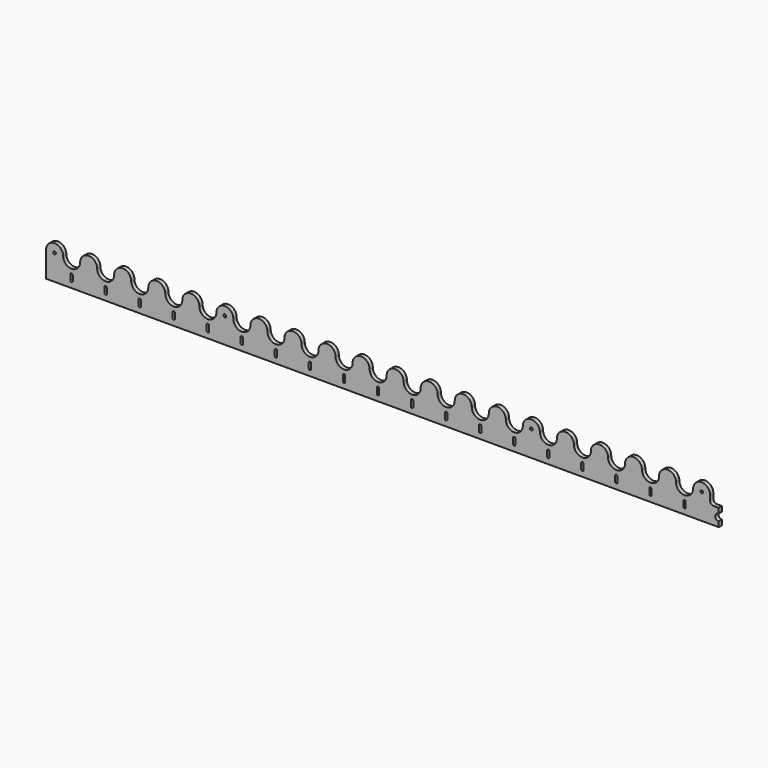
from build123d import *

# Parameters (mm, degrees)
F0_R     = 4
F1_DEPTH = 12


# Not quite as in the source:
# - ends of sketch curves that miss each other by under 0.0002 mm in the source are joined


with BuildPart() as f1:
    # F0 (on Front) → F1 (new body)
    with BuildSketch(Plane.XZ):
        with BuildLine():
            ThreePointArc((91.0431935055, 71.2102863897), (66.0431935055, 96.2102863897), (41.0431935055, 71.2102863897))
            ThreePointArc((41.0431935055, 71.2102863897), (16.0431935055, 46.2102863897), (-8.9568064945, 71.2102863897))
            ThreePointArc((-8.9568064945, 71.2102863897), (-33.9568064945, 96.2102863897), (-58.9568064945, 71.2102863897))
            Line((-58.9568064945, 71.2102863897), (-58.9568064945, -3.7897136103))
            Line((-58.9568064945, -3.7897136103), (1891.0431935055, -3.7897136103))
            Line((1891.0431935055, -3.7897136103), (1916.0431861877, -3.7897136103))
            Line((1916.0431861877, -3.7897136103), (1916.0431861877, 11.2232529739))
            ThreePointArc((1916.0431861877, 11.2232529739), (1906.0431861877, 21.2232529739), (1916.0431861877, 31.2232529739))
            Line((1916.0431861877, 31.2232529739), (1916.0431861877, 46.2362195582))
            Line((1916.0431861877, 46.2362195582), (1901.0431884565, 46.2362195582))
            ThreePointArc((1901.0431884565, 46.2362195582), (1893.9756743288, 49.1615998472), (1891.0431935055, 56.2261707472))
            Line((1891.0431935055, 56.2261707472), (1891.0431935055, 56.4615577459))
            Line((1891.0431935055, 56.4615577459), (1891.0431935055, 71.2102863897))
            ThreePointArc((1891.0431935055, 71.2102863897), (1866.0431935055, 96.2102863897), (1841.0431935055, 71.2102863897))
            ThreePointArc((1841.0431935055, 71.2102863897), (1816.0431935055, 46.2102863897), (1791.0431935055, 71.2102863897))
            ThreePointArc((1791.0431935055, 71.2102863897), (1766.0431935055, 96.2102863897), (1741.0431935055, 71.2102863897))
            ThreePointArc((1741.0431935055, 71.2102863897), (1716.0431935055, 46.2102863897), (1691.0431935055, 71.2102863897))
            ThreePointArc((1691.0431935055, 71.2102863897), (1666.0431935055, 96.2102863897), (1641.0431935055, 71.2102863897))
            ThreePointArc((1641.0431935055, 71.2102863897), (1616.0431935055, 46.2102863897), (1591.0431935055, 71.2102863897))
            ThreePointArc((1591.0431935055, 71.2102863897), (1566.0431935055, 96.2102863897), (1541.0431935055, 71.2102863897))
            ThreePointArc((1541.0431935055, 71.2102863897), (1516.0431935055, 46.2102863897), (1491.0431935055, 71.2102863897))
            ThreePointArc((1491.0431935055, 71.2102863897), (1466.0431935055, 96.2102863897), (1441.0431935055, 71.2102863897))
            ThreePointArc((1441.0431935055, 71.2102863897), (1416.0431935055, 46.2102863897), (1391.0431935055, 71.2102863897))
            ThreePointArc((1391.0431935055, 71.2102863897), (1366.0431935055, 96.2102863897), (1341.0431935055, 71.2102863897))
            ThreePointArc((1341.0431935055, 71.2102863897), (1316.0431935055, 46.2102863897), (1291.0431935055, 71.2102863897))
            ThreePointArc((1291.0431935055, 71.2102863897), (1266.0431935055, 96.2102863897), (1241.0431935055, 71.2102863897))
            ThreePointArc((1241.0431935055, 71.2102863897), (1216.0431935055, 46.2102863897), (1191.0431935055, 71.2102863897))
            ThreePointArc((1191.0431935055, 71.2102863897), (1166.0431935055, 96.2102863897), (1141.0431935055, 71.2102863897))
            ThreePointArc((1141.0431935055, 71.2102863897), (1116.0431935055, 46.2102863897), (1091.0431935055, 71.2102863897))
            ThreePointArc((1091.0431935055, 71.2102863897), (1066.0431935055, 96.2102863897), (1041.0431935055, 71.2102863897))
            ThreePointArc((1041.0431935055, 71.2102863897), (1016.0431935055, 46.2102863897), (991.0431935055, 71.2102863897))
            ThreePointArc((991.0431935055, 71.2102863897), (966.0431935055, 96.2102863897), (941.0431935055, 71.2102863897))
            ThreePointArc((941.0431935055, 71.2102863897), (916.0431935055, 46.2102863897), (891.0431935055, 71.2102863897))
            ThreePointArc((891.0431935055, 71.2102863897), (866.0431935055, 96.2102863897), (841.0431935055, 71.2102863897))
            ThreePointArc((841.0431935055, 71.2102863897), (816.0431935055, 46.2102863897), (791.0431935055, 71.2102863897))
            ThreePointArc((791.0431935055, 71.2102863897), (766.0431935055, 96.2102863897), (741.0431935055, 71.2102863897))
            ThreePointArc((741.0431935055, 71.2102863897), (716.0431935055, 46.2102863897), (691.0431935055, 71.2102863897))
            ThreePointArc((691.0431935055, 71.2102863897), (666.0431935055, 96.2102863897), (641.0431935055, 71.2102863897))
            ThreePointArc((641.0431935055, 71.2102863897), (616.0431935055, 46.2102863897), (591.0431935055, 71.2102863897))
            ThreePointArc((591.0431935055, 71.2102863897), (566.0431935055, 96.2102863897), (541.0431935055, 71.2102863897))
            ThreePointArc((541.0431935055, 71.2102863897), (516.0431935055, 46.2102863897), (491.0431935055, 71.2102863897))
            ThreePointArc((491.0431935055, 71.2102863897), (466.0431935055, 96.2102863897), (441.0431935055, 71.2102863897))
            ThreePointArc((441.0431935055, 71.2102863897), (416.0431935055, 46.2102863897), (391.0431935055, 71.2102863897))
            ThreePointArc((391.0431935055, 71.2102863897), (366.0431935055, 96.2102863897), (341.0431935055, 71.2102863897))
            ThreePointArc((341.0431935055, 71.2102863897), (316.0431935055, 46.2102863897), (291.0431935055, 71.2102863897))
            ThreePointArc((291.0431935055, 71.2102863897), (266.0431935055, 96.2102863897), (241.0431935055, 71.2102863897))
            ThreePointArc((241.0431935055, 71.2102863897), (216.0431935055, 46.2102863897), (191.0431935055, 71.2102863897))
            ThreePointArc((191.0431935055, 71.2102863897), (166.0431935055, 96.2102863897), (141.0431935055, 71.2102863897))
            ThreePointArc((141.0431935055, 71.2102863897), (116.0431935055, 46.2102863897), (91.0431935055, 71.2102863897))
        make_face()
        with BuildLine():
            ThreePointArc((12.3674108083, 31.0259666217), (15.8490323457, 34.5622976712), (19.3672217487, 31.0623449364))
            Line((19.3672217487, 31.0623449364), (19.3672217487, 14.9847705892))
            ThreePointArc((19.3672217487, 14.9847705892), (15.8854111516, 11.4848178545), (12.3674108083, 14.9483922746))
            Line((12.3674108083, 14.9483922746), (12.3674108083, 31.0259666217))
        make_face(mode=Mode.SUBTRACT)
        with BuildLine():
            Line((112.3674108083, 14.9483922746), (112.3674108083, 31.0259666217))
            ThreePointArc((112.3674108083, 31.0259666217), (115.8490323457, 34.5622976712), (119.3672217487, 31.0623449364))
            Line((119.3672217487, 31.0623449364), (119.3672217487, 14.9847705892))
            ThreePointArc((119.3672217487, 14.9847705892), (115.8854111516, 11.4848178545), (112.3674108083, 14.9483922746))
        make_face(mode=Mode.SUBTRACT)
        with BuildLine():
            Line((212.3674108083, 14.9483922746), (212.3674108083, 31.0259666217))
            ThreePointArc((212.3674108083, 31.0259666217), (215.8490323457, 34.5622976712), (219.3672217487, 31.0623449364))
            Line((219.3672217487, 31.0623449364), (219.3672217487, 14.9847705892))
            ThreePointArc((219.3672217487, 14.9847705892), (215.8854111516, 11.4848178545), (212.3674108083, 14.9483922746))
        make_face(mode=Mode.SUBTRACT)
        with BuildLine():
            Line((312.3674108083, 14.9483922746), (312.3674108083, 31.0259666217))
            ThreePointArc((312.3674108083, 31.0259666217), (315.8490323457, 34.5622976712), (319.3672217487, 31.0623449364))
            Line((319.3672217487, 31.0623449364), (319.3672217487, 14.9847705892))
            ThreePointArc((319.3672217487, 14.9847705892), (315.8854111516, 11.4848178545), (312.3674108083, 14.9483922746))
        make_face(mode=Mode.SUBTRACT)
        with BuildLine():
            Line((412.3674108083, 14.9483922746), (412.3674108083, 31.0259666217))
            ThreePointArc((412.3674108083, 31.0259666217), (415.8490323457, 34.5622976712), (419.3672217487, 31.0623449364))
            Line((419.3672217487, 31.0623449364), (419.3672217487, 14.9847705892))
            ThreePointArc((419.3672217487, 14.9847705892), (415.8854111516, 11.4848178545), (412.3674108083, 14.9483922746))
        make_face(mode=Mode.SUBTRACT)
        with BuildLine():
            Line((512.3674108083, 14.9483922746), (512.3674108083, 31.0259666217))
            ThreePointArc((512.3674108083, 31.0259666217), (515.8490323457, 34.5622976712), (519.3672217487, 31.0623449364))
            Line((519.3672217487, 31.0623449364), (519.3672217487, 14.9847705892))
            ThreePointArc((519.3672217487, 14.9847705892), (515.8854111516, 11.4848178545), (512.3674108083, 14.9483922746))
        make_face(mode=Mode.SUBTRACT)
        with BuildLine():
            Line((612.3674108083, 14.9483922746), (612.3674108083, 31.0259666217))
            ThreePointArc((612.3674108083, 31.0259666217), (615.8490323457, 34.5622976712), (619.3672217487, 31.0623449364))
            Line((619.3672217487, 31.0623449364), (619.3672217487, 14.9847705892))
            ThreePointArc((619.3672217487, 14.9847705892), (615.8854111516, 11.4848178545), (612.3674108083, 14.9483922746))
        make_face(mode=Mode.SUBTRACT)
        with BuildLine():
            Line((712.3674108083, 14.9483922746), (712.3674108083, 31.0259666217))
            ThreePointArc((712.3674108083, 31.0259666217), (715.8490323457, 34.5622976712), (719.3672217487, 31.0623449364))
            Line((719.3672217487, 31.0623449364), (719.3672217487, 14.9847705892))
            ThreePointArc((719.3672217487, 14.9847705892), (715.8854111516, 11.4848178545), (712.3674108083, 14.9483922746))
        make_face(mode=Mode.SUBTRACT)
        with BuildLine():
            Line((812.3674108083, 14.9483922746), (812.3674108083, 31.0259666217))
            ThreePointArc((812.3674108083, 31.0259666217), (815.8490323457, 34.5622976712), (819.3672217487, 31.0623449364))
            Line((819.3672217487, 31.0623449364), (819.3672217487, 14.9847705892))
            ThreePointArc((819.3672217487, 14.9847705892), (815.8854111516, 11.4848178545), (812.3674108083, 14.9483922746))
        make_face(mode=Mode.SUBTRACT)
        with BuildLine():
            Line((912.3674108083, 14.9483922746), (912.3674108083, 31.0259666217))
            ThreePointArc((912.3674108083, 31.0259666217), (915.8490323457, 34.5622976712), (919.3672217487, 31.0623449364))
            Line((919.3672217487, 31.0623449364), (919.3672217487, 14.9847705892))
            ThreePointArc((919.3672217487, 14.9847705892), (915.8854111516, 11.4848178545), (912.3674108083, 14.9483922746))
        make_face(mode=Mode.SUBTRACT)
        with BuildLine():
            Line((1012.3674108083, 14.9483922746), (1012.3674108083, 31.0259666217))
            ThreePointArc((1012.3674108083, 31.0259666217), (1015.8490323457, 34.5622976712), (1019.3672217487, 31.0623449364))
            Line((1019.3672217487, 31.0623449364), (1019.3672217487, 14.9847705892))
            ThreePointArc((1019.3672217487, 14.9847705892), (1015.8854111516, 11.4848178545), (1012.3674108083, 14.9483922746))
        make_face(mode=Mode.SUBTRACT)
        with BuildLine():
            Line((1112.3674108083, 14.9483922746), (1112.3674108083, 31.0259666217))
            ThreePointArc((1112.3674108083, 31.0259666217), (1115.8490323457, 34.5622976712), (1119.3672217487, 31.0623449364))
            Line((1119.3672217487, 31.0623449364), (1119.3672217487, 14.9847705892))
            ThreePointArc((1119.3672217487, 14.9847705892), (1115.8854111516, 11.4848178545), (1112.3674108083, 14.9483922746))
        make_face(mode=Mode.SUBTRACT)
        with BuildLine():
            Line((1212.3674108083, 14.9483922746), (1212.3674108083, 31.0259666217))
            ThreePointArc((1212.3674108083, 31.0259666217), (1215.8490323457, 34.5622976712), (1219.3672217487, 31.0623449364))
            Line((1219.3672217487, 31.0623449364), (1219.3672217487, 14.9847705892))
            ThreePointArc((1219.3672217487, 14.9847705892), (1215.8854111516, 11.4848178545), (1212.3674108083, 14.9483922746))
        make_face(mode=Mode.SUBTRACT)
        with BuildLine():
            Line((1312.3674108083, 14.9483922746), (1312.3674108083, 31.0259666217))
            ThreePointArc((1312.3674108083, 31.0259666217), (1315.8490323457, 34.5622976712), (1319.3672217487, 31.0623449364))
            Line((1319.3672217487, 31.0623449364), (1319.3672217487, 14.9847705892))
            ThreePointArc((1319.3672217487, 14.9847705892), (1315.8854111516, 11.4848178545), (1312.3674108083, 14.9483922746))
        make_face(mode=Mode.SUBTRACT)
        with BuildLine():
            Line((1412.3674108083, 14.9483922746), (1412.3674108083, 31.0259666217))
            ThreePointArc((1412.3674108083, 31.0259666217), (1415.8490323457, 34.5622976712), (1419.3672217487, 31.0623449364))
            Line((1419.3672217487, 31.0623449364), (1419.3672217487, 14.9847705892))
            ThreePointArc((1419.3672217487, 14.9847705892), (1415.8854111516, 11.4848178545), (1412.3674108083, 14.9483922746))
        make_face(mode=Mode.SUBTRACT)
        with BuildLine():
            Line((1512.3674108083, 14.9483922746), (1512.3674108083, 31.0259666217))
            ThreePointArc((1512.3674108083, 31.0259666217), (1515.8490323457, 34.5622976712), (1519.3672217487, 31.0623449364))
            Line((1519.3672217487, 31.0623449364), (1519.3672217487, 14.9847705892))
            ThreePointArc((1519.3672217487, 14.9847705892), (1515.8854111516, 11.4848178545), (1512.3674108083, 14.9483922746))
        make_face(mode=Mode.SUBTRACT)
        with BuildLine():
            Line((1612.3674108083, 14.9483922746), (1612.3674108083, 31.0259666217))
            ThreePointArc((1612.3674108083, 31.0259666217), (1615.8490323457, 34.5622976712), (1619.3672217487, 31.0623449364))
            Line((1619.3672217487, 31.0623449364), (1619.3672217487, 14.9847705892))
            ThreePointArc((1619.3672217487, 14.9847705892), (1615.8854111516, 11.4848178545), (1612.3674108083, 14.9483922746))
        make_face(mode=Mode.SUBTRACT)
        with BuildLine():
            Line((1712.3674108083, 14.9483922746), (1712.3674108083, 31.0259666217))
            ThreePointArc((1712.3674108083, 31.0259666217), (1715.8490323457, 34.5622976712), (1719.3672217487, 31.0623449364))
            Line((1719.3672217487, 31.0623449364), (1719.3672217487, 14.9847705892))
            ThreePointArc((1719.3672217487, 14.9847705892), (1715.8854111516, 11.4848178545), (1712.3674108083, 14.9483922746))
        make_face(mode=Mode.SUBTRACT)
        with BuildLine():
            Line((1812.3674108083, 14.9483922746), (1812.3674108083, 31.0259666217))
            ThreePointArc((1812.3674108083, 31.0259666217), (1815.8490323457, 34.5622976712), (1819.3672217487, 31.0623449364))
            Line((1819.3672217487, 31.0623449364), (1819.3672217487, 14.9847705892))
            ThreePointArc((1819.3672217487, 14.9847705892), (1815.8854111516, 11.4848178545), (1812.3674108083, 14.9483922746))
        make_face(mode=Mode.SUBTRACT)
        with Locations((466.0431935055, 71.2102863897)):
            Circle(F0_R, mode=Mode.SUBTRACT)
        with Locations((-33.9568064945, 71.2102863897)):
            Circle(F0_R, mode=Mode.SUBTRACT)
        with Locations((1366.0431935055, 71.2102863897)):
            Circle(F0_R, mode=Mode.SUBTRACT)
        with Locations((1866.0431935055, 71.2102863897)):
            Circle(F0_R, mode=Mode.SUBTRACT)
    extrude(amount=F1_DEPTH)


solid = f1.part
